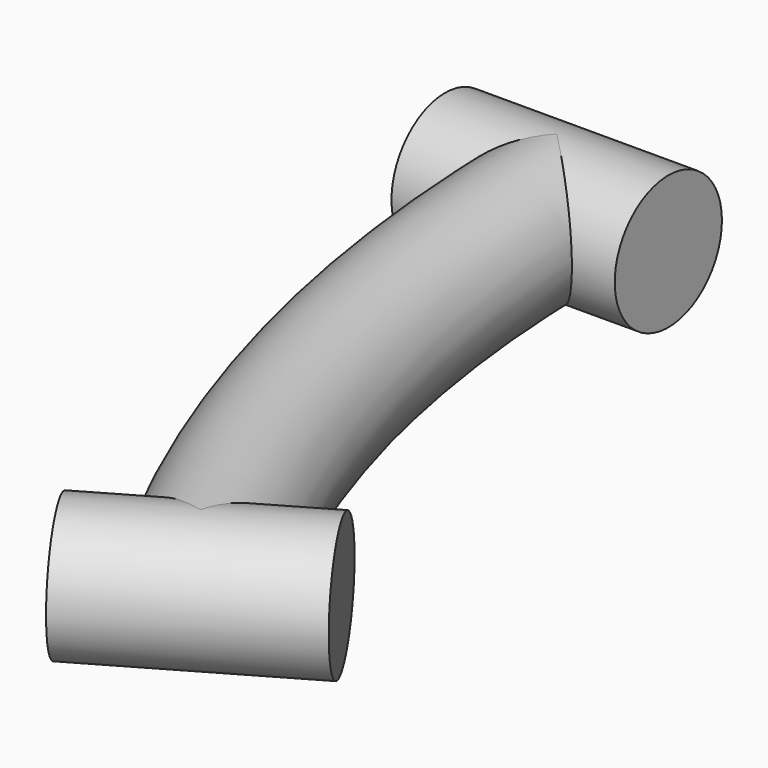
from build123d import *

# Parameters (mm, degrees)
F0_R     = 3.81
F3_R     = 3.81
F4_DEPTH = 6.35
F7_R     = 3.81
F8_DEPTH = 6.35


with BuildPart() as f2:
    # F2: sweep along a path in F1
    with BuildLine(Plane.XY) as f2_path:
        ThreePointArc((0, 0), (2.5964520368, -19.7220112368), (10.2088642316, -38.1))
    # F0 (on Front) → F2 (sweep)
    with BuildSketch(Plane.XZ):
        Circle(F0_R)
    sweep(path=f2_path.line)

    # F3 (on Right) → F4 (join, symmetric)
    with BuildSketch(Plane.YZ):
        Circle(F3_R)
    extrude(amount=F4_DEPTH, both=True)

    # F7 (on face) → F8 (join, symmetric)
    with BuildSketch(Plane(origin=(-8.8411357684, -5.1044321158, 0), x_dir=(-0.5, 0.8660254038, 0), z_dir=(0.8660254038, 0.5, 0))):
        with Locations((-38.1, 0)):
            Circle(F7_R)
    extrude(amount=F8_DEPTH, both=True)


solid = f2.part
